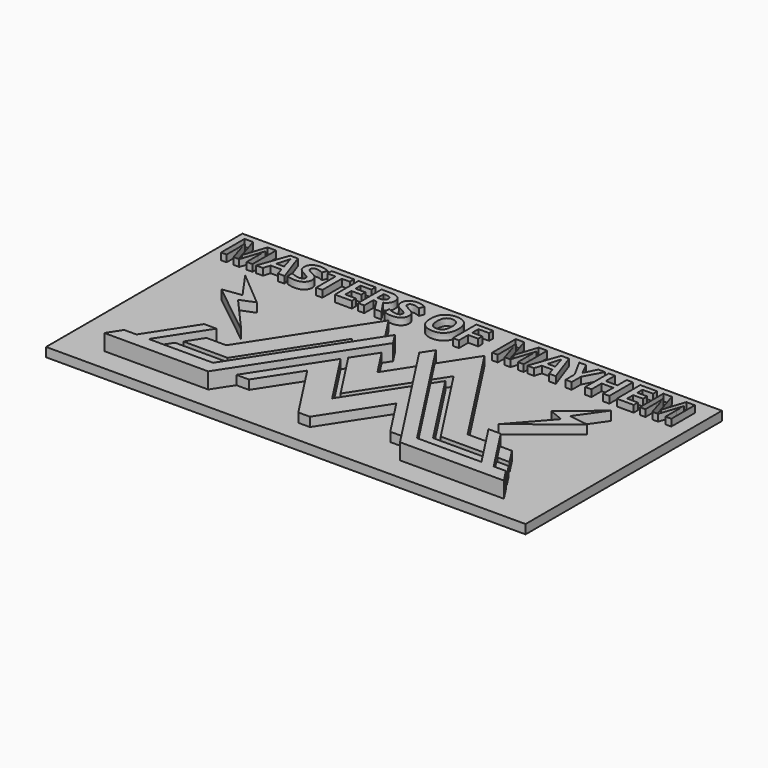
from build123d import *

# Parameters (mm, degrees)
F7_DEPTH      = 2.032
F8_DEPTH      = 2.032
F9_DEPTH      = 3.556
F6_W          = 106.68
F6_H          = 54.61
F10_DEPTH     = 2.032
F11_TEXT_SIZE = 9.1722222222
F13_TEXT_SIZE = 9.1722222222
F12_TEXT_SIZE = 9.1722222222
F14_DEPTH     = 1.524
F16_DEPTH     = 2.032


# Not quite as in the source:
# - Text() gives the source's letters only with a copy of the font that has no kerning and outlines rounded to 1/6400 em; it was checked with that copy


with BuildPart() as f7:
    # F2 (on offset) → F7 (new body)
    with BuildSketch(Plane.XY.offset(2.032)):
        Polygon((10.668, 36.83), (0, 20.402720566), (-10.668, 36.83), (-26.8425561134, 11.9233677358), (-36.7068744559, 11.9233677358), (-39.0161678573, 8.3673677358), (-23.7003645399, 8.3673677358), (-11.2737205528, 27.5027214294), (0, 10.1427141384), (11.2737205528, 27.5027214294), (23.7003645399, 8.3673677358), (39.0161678573, 8.3673677358), (36.7068744559, 11.9233677358), (26.8425561134, 11.9233677358), align=None)
    extrude(amount=F7_DEPTH)



with BuildPart() as f8:
    # F5 (on offset) → F8 (new body)
    with BuildSketch(Plane.XY.offset(2.032)):
        Polygon((23.0108108014, 7.0973677358), (11.2737205528, 25.1709017868), (0, 7.8108944957), (-11.2737205528, 25.1709017868), (-23.0108108014, 7.0973677358), (-39.8409155007, 7.0973677358), (-41.6458580126, 4.318), (-24.8157533133, 4.318), (-15.7202464038, 4.318), (-9.906, 13.2711543282), (-1.2876116088, 0), (0, 0), (1.2876116088, 0), (9.906, 13.2711543282), (15.7202464038, 4.318), (24.8157533133, 4.318), (41.6458580126, 4.318), (39.8409155007, 7.0973677358), align=None)
    extrude(amount=F8_DEPTH)


with BuildPart() as f7_1:
    add(f7.part)

    add(f8.part)  # F9 merges F8
    # F3 (on offset) → F9 (join)
    with BuildSketch(Plane.XY.offset(2.032)):
        Polygon((-21.336, 0), (-2.9062684799, 28.3792978603), (-4.572, 30.9442994672), (-22.6880686961, 3.048), (-37.0191206811, 3.048), (-30.265692309, 13.4473677358), (-32.9914347964, 13.4473677358), (-39.7448631685, 3.048), (-42.4706056559, 3.048), (-44.45, 0), align=None)
        Polygon((21.336, 0), (44.45, 0), (42.4706056559, 3.048), (39.7448631685, 3.048), (32.9914347964, 13.4473677358), (30.265692309, 13.4473677358), (37.0191206811, 3.048), (22.6880686961, 3.048), (4.572, 30.9442994672), (2.9062684799, 28.3792978603), align=None)
    extrude(amount=F9_DEPTH)

    # F6 (on Top) → F10 (join)
    with BuildSketch(Plane.XY):
        with Locations((0, 22.225)):
            Rectangle(F6_W, F6_H)
    extrude(amount=F10_DEPTH)

    # F11 (on offset) + F13 (on offset) + F12 (on offset) → F14 (join)
    with BuildSketch(Plane.XY.offset(2.032)):
        with Locations((-50.8, 39.37)):
            Text('MASTERS', F11_TEXT_SIZE, font='Open Sans', font_style=FontStyle.BOLD, text_align=(TextAlign.LEFT, TextAlign.BOTTOM))
    with BuildSketch(Plane.XY.offset(2.032)):
        with Locations((-6.5333585185, 39.37)):
            Text('OF', F13_TEXT_SIZE, font='Open Sans', font_style=FontStyle.BOLD, text_align=(TextAlign.LEFT, TextAlign.BOTTOM))
    with BuildSketch(Plane.XY.offset(2.032)):
        with Locations((9.5264331597, 39.37)):
            Text('MAYHEM', F12_TEXT_SIZE, font='Open Sans', font_style=FontStyle.BOLD, text_align=(TextAlign.LEFT, TextAlign.BOTTOM))
    extrude(amount=F14_DEPTH)

    # F15 (on offset) → F16 (join)
    with BuildSketch(Plane.XY.offset(2.032)):
        Polygon((36.429900676, 28.4173302352), (40.7001823187, 34.4922244549), (32.7868318757, 27.8283506632), (35.9390862286, 26.5522282571), (28.6159794778, 18.2564724237), (40.6805361875, 27.8283506632), align=None)
        Polygon((-32.7868318757, 27.8283506632), (-40.7001823187, 34.4922244549), (-36.429900676, 28.4173302352), (-40.6805361875, 27.8283506632), (-28.6159794778, 18.2564724237), (-35.9390862286, 26.5522282571), align=None)
    extrude(amount=F16_DEPTH)


solid = f7_1.part
